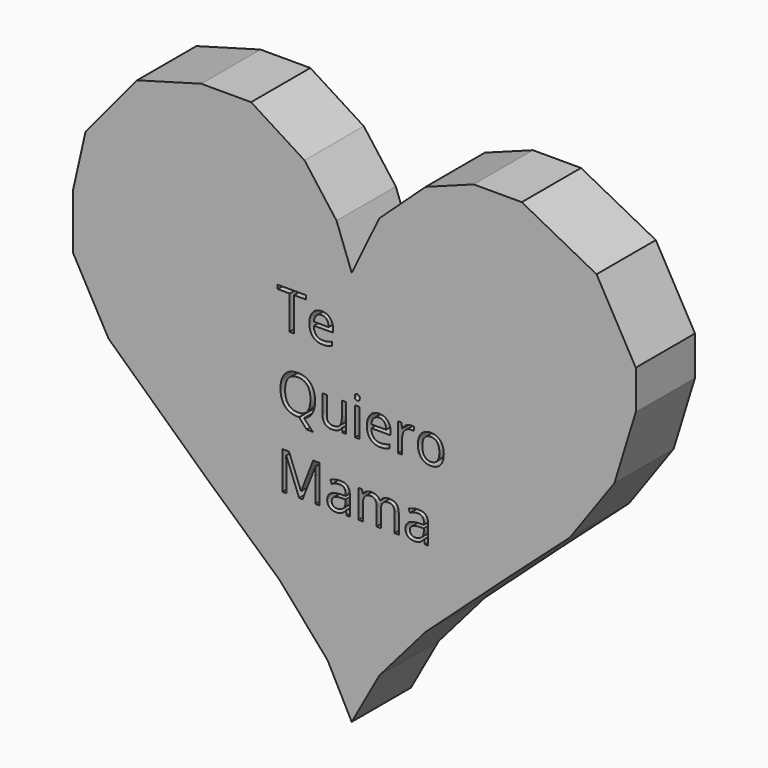
from build123d import *

# Parameters (mm, degrees)
F1_DEPTH     = 12.7
F2_TEXT_SIZE = 9.0277777778
F3_DEPTH     = 12.701


# Not quite as in the source:
# - Text() gives the source's letters only with a copy of the font that has no kerning and outlines rounded to 1/6400 em; it was checked with that copy


with BuildPart() as f1:
    # F0 (on Front) → F1 (new body)
    with BuildSketch(Plane.XZ):
        Polygon((4.7334171832, 30.0800967962), (0, 20.3078817576), (-2.5957447942, 27.3316595703), (-8.0926157534, 34.6608199179), (-17.2540657222, 40.4630750418), (-25.804752484, 40.4630750418), (-36.798492074, 37.4092571437), (-45.6545613706, 26.7208982259), (-47.7922335267, 17.2540657222), (-47.7922335267, 7.7872332186), (-41.6845977306, -3.2065075357), (-24.888606742, -18.7809728086), (-12.367958203, -30.0800967962), (-4.1226525791, -39.5469255745), (0, -47.4868528545), (4.7334171832, -38.9361642301), (12.6733388752, -29.7747142613), (25.8047506213, -17.8648289293), (37.4092571437, -7.4818511494), (45.0438000262, 3.2065075357), (48.7083792686, 15.1163935661), (48.7083792686, 21.8347907066), (41.9899821281, 33.7446779013), (29.1639491916, 40.4630750418), (20.9186449647, 40.4630750418), (12.6733388752, 37.4092571437), align=None)
    extrude(amount=F1_DEPTH)

    # F2 (on Front) → F3 (cut, through all)
    with BuildSketch(Plane.XZ):
        with Locations((-12.7622109644, 7.9426539022)):
            Text('Te', F2_TEXT_SIZE, font='Open Sans', text_align=(TextAlign.LEFT, TextAlign.BOTTOM))
        with Locations((-12.7622109644, -4.3351238756)):
            Text('Quiero', F2_TEXT_SIZE, font='Open Sans', text_align=(TextAlign.LEFT, TextAlign.BOTTOM))
        with Locations((-12.7622109644, -16.6129016534)):
            Text('Mama', F2_TEXT_SIZE, font='Open Sans', text_align=(TextAlign.LEFT, TextAlign.BOTTOM))
    extrude(amount=F3_DEPTH, mode=Mode.SUBTRACT)


solid = f1.part
